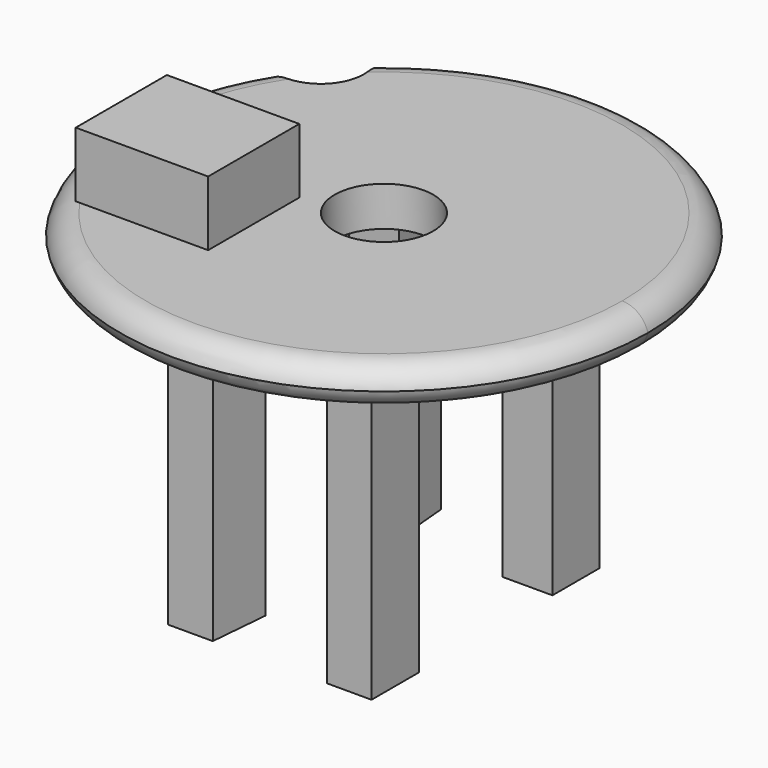
from build123d import *

# Parameters (mm, degrees)
F1_DEPTH    = 7.62
F3_DEPTH    = 57.15
F4_T2_ANGLE = 118.6593978475
F4_T4_ANGLE = 118.6593978475
F7_R        = 8.2517563721
F8_DEPTH    = 25.4
F9_R        = 9.4542856314
F10_DEPTH   = 26.162
F11_W       = 25.4
F11_H       = 21.8551358064
F12_DEPTH   = 12.446


# Not quite as in the source:
# - a fillet or chamfer that OpenCascade refuses, or shapes differently, is made with other operations: its cross-section is extruded or revolved along the edge and cut away or added


with BuildPart() as f1:
    # F0 (on Top) → F1 (new body)
    with BuildSketch(Plane.XY):
        with BuildLine():
            ThreePointArc((0, -50.8), (35.9210244843, -35.9210244843), (50.8, 0))
            Line((50.8, 0), (0, 0))
            Line((0, 0), (0, -50.8))
        make_face()
    extrude(amount=F1_DEPTH)

    # F2 (on face) → F3 (join)
    with BuildSketch(Plane(origin=(0, 0, 0), x_dir=(1, 0, 0), z_dir=(0, 0, -1))):
        Polygon((19.5075478405, 27.366604656), (10.9492652118, 27.366604656), (9.9541153759, 16.0219036043), (19.5075478405, 16.0219036043), align=None)
    extrude(amount=F3_DEPTH)

    # F4: fillet of radius 5.08 on 2 edges, made by hand

    # F4_s1 → F4_t2 (revolve, cut)
    with BuildSketch(Plane(origin=(0, 0, 0), x_dir=(0, 0, 1), z_dir=(-0.9688875708, 0.247501263, 0))):
        with BuildLine():
            ThreePointArc((2.54, -50.8), (6.1321024484, -49.3121024484), (7.62, -45.72))
            Line((7.62, -45.72), (7.62, -50.8))
            Line((7.62, -50.8), (2.54, -50.8))
        make_face()
    revolve(axis=Axis((0, 0, 7.62), (0, 0, 1)), revolution_arc=F4_T2_ANGLE, mode=Mode.SUBTRACT)

    # F4_s3 → F4_t4 (revolve, cut)
    with BuildSketch(Plane(origin=(0, 0, 0), x_dir=(0, 0, 1), z_dir=(-0.9688875708, 0.247501263, 0))):
        with BuildLine():
            ThreePointArc((5.08, -50.8), (1.4878975516, -49.3121024484), (0, -45.72))
            Line((0, -45.72), (0, -50.8))
            Line((0, -50.8), (5.08, -50.8))
        make_face()
    revolve(axis=Axis((0, 0, 0), (0, 0, 1)), revolution_arc=F4_T4_ANGLE, mode=Mode.SUBTRACT)

    # F5: F1 across plane


with BuildPart() as f1_1:
    add(f1.part)
    add(f1.part.mirror(Plane.YZ))

    # F6: F1 across plane


with BuildPart() as f1_2:
    add(f1_1.part)
    add(f1_1.part.mirror(Plane.XZ))

    # F7 (on face) → F8 (cut)
    with BuildSketch(Plane.XY.offset(7.62)):
        with Locations((-38.7037992477, 33.2289077342)):
            Circle(F7_R)
    extrude(amount=-F8_DEPTH, mode=Mode.SUBTRACT)

    # F9 (on face) → F10 (cut)
    with BuildSketch(Plane.XY.offset(7.62)):
        Circle(F9_R)
    extrude(amount=-F10_DEPTH, mode=Mode.SUBTRACT)

    # F11 (on face) → F12 (join)
    with BuildSketch(Plane.XY.offset(7.62)):
        with Locations((-25.7072858512, -14.9798975326)):
            Rectangle(F11_W, F11_H)
    extrude(amount=F12_DEPTH)


solid = f1_2.part
